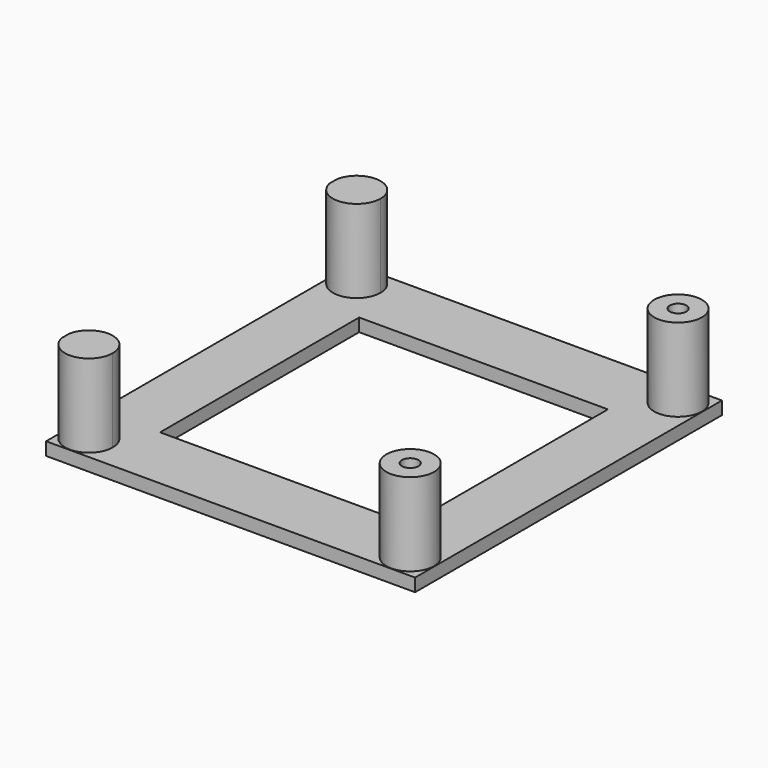
from build123d import *

# Parameters (mm, degrees)
F0_W     = 45.212
F0_H     = 46.99
F1_DEPTH = 1.5875
F2_W     = 30.48
F2_H     = 30.48
F3_DEPTH = 6.35
F4_R     = 2.921
F4_R_2   = 1.016
F5_DEPTH = 10.16
F6_DEPTH = 6.35


with BuildPart() as f1:
    # F0 (on Top) → F1 (new body)
    with BuildSketch(Plane.XY):
        Rectangle(F0_W, F0_H)
    extrude(amount=F1_DEPTH)

    # F2 (on face) → F3 (cut)
    with BuildSketch(Plane.XY.offset(1.5875)):
        Rectangle(F2_W, F2_H)
    extrude(amount=-F3_DEPTH, mode=Mode.SUBTRACT)

    # F4 (on face) → F5 (join)
    with BuildSketch(Plane.XY.offset(1.5875)):
        with Locations((19.6215, -20.5105)):
            Circle(F4_R)
        with Locations((19.6215, -20.5105)):
            Circle(F4_R_2, mode=Mode.SUBTRACT)
        with BuildLine():
            ThreePointArc((-22.606, 19.9047486071), (-19.4439646983, 17.6054183746), (-16.8275, 20.5105))
            ThreePointArc((-16.8275, 20.5105), (-19.4439646983, 23.4155816254), (-22.606, 21.1162513929))
            Line((-22.606, 21.1162513929), (-22.606, 19.9047486071))
        make_face()
        with BuildLine():
            ThreePointArc((-16.8275, -20.5105), (-19.4439646983, -17.6054183746), (-22.606, -19.9047486071))
            Line((-22.606, -19.9047486071), (-22.606, -21.1162513929))
            ThreePointArc((-22.606, -21.1162513929), (-19.4439646983, -23.4155816254), (-16.8275, -20.5105))
        make_face()
        with Locations((19.6215, 20.5105)):
            Circle(F4_R)
        with Locations((19.6215, 20.5105)):
            Circle(F4_R_2, mode=Mode.SUBTRACT)
    extrude(amount=F5_DEPTH)

    # F4 (on face) → F6 (cut)
    with BuildSketch(Plane.XY.offset(1.5875)):
        with Locations((19.6215, -20.5105)):
            Circle(F4_R_2)
        with Locations((19.6215, 20.5105)):
            Circle(F4_R_2)
    extrude(amount=-F6_DEPTH, mode=Mode.SUBTRACT)


solid = f1.part
